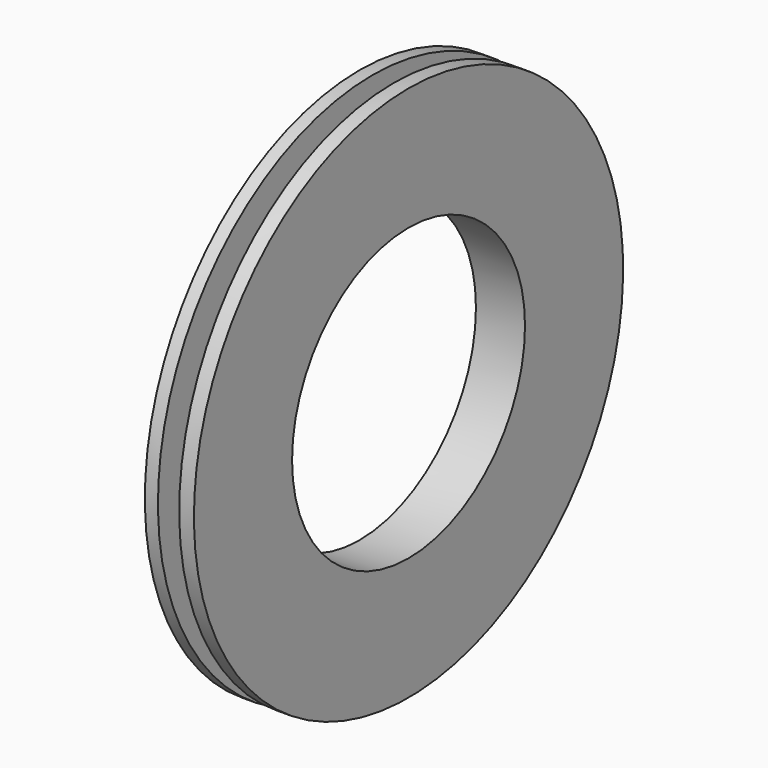
from build123d import *

# Parameters (mm, degrees)
F0_W   = 8
F0_H   = 8.5
F0_W_2 = 13
F0_H_2 = 11.5
F0_W_3 = 9


with BuildPart() as f1:
    # F0 (on Front) → F1 (revolve)
    with BuildSketch(Plane.XZ):
        Polygon((0, 164), (0, 97.5), (8, 97.5), (8, 109), (8, 164), align=None)
        with Locations((4, 93.25)):
            Rectangle(F0_W, F0_H)
        Polygon((21, 109), (21, 97.5), (30, 97.5), (30, 164), (21, 164), align=None)
        with Locations((14.5, 103.25)):
            Rectangle(F0_W_2, F0_H_2)
        with Locations((14.5, 93.25)):
            Rectangle(F0_W_2, F0_H)
        with Locations((25.5, 93.25)):
            Rectangle(F0_W_3, F0_H)
    revolve(axis=Axis((49, 0, 0), (1, 0, 0)))


solid = f1.part
